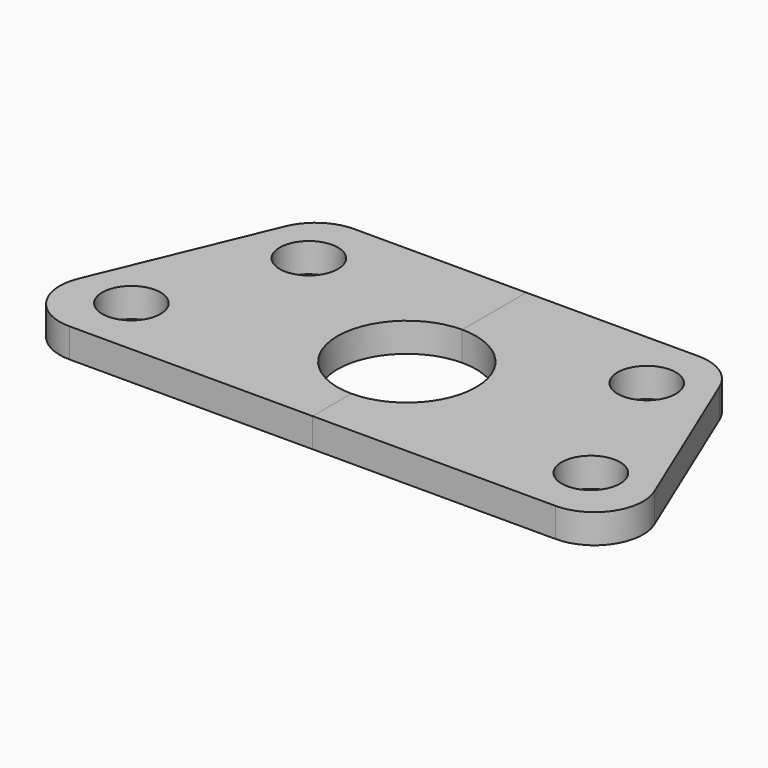
from build123d import *
from build123d import SkipClean  # not in build123d's __all__

# Parameters (mm, degrees)
F0_R     = 6
F1_DEPTH = 6


with BuildPart() as f1:
    # F0 (on Top) → F1 (new body)
    with BuildSketch(Plane.XY):
        with BuildLine():
            Line((0, -16.5), (0, 0))
            Line((0, 0), (-35.4166666667, 0))
            ThreePointArc((-35.4166666667, 0), (-40.9636686289, -1.6794970566), (-44.6474358974, -6.1538461538))
            Line((-44.6474358974, -6.1538461538), (-59.2307692308, -41.1538461538))
            ThreePointArc((-59.2307692308, -41.1538461538), (-58.3205029434, -50.5470019623), (-50, -55))
            Line((-50, -55), (0, -55))
            Line((0, -55), (0, -45))
            ThreePointArc((0, -45), (-14.25, -30.75), (0, -16.5))
        make_face()
        with Locations((-47.25, -42.5)):
            Circle(F0_R, mode=Mode.SUBTRACT)
        with Locations((-34.75, -12.5)):
            Circle(F0_R, mode=Mode.SUBTRACT)
    extrude(amount=F1_DEPTH)

    # F2: F1 across plane


with BuildPart() as f1_1:
    add(f1.part, clean=False)
    with SkipClean():  # cleaning this boolean's faces spoils the solid; the shape is the same uncleaned
        add(f1.part.mirror(Plane.YZ), clean=False)


solid = f1_1.part
